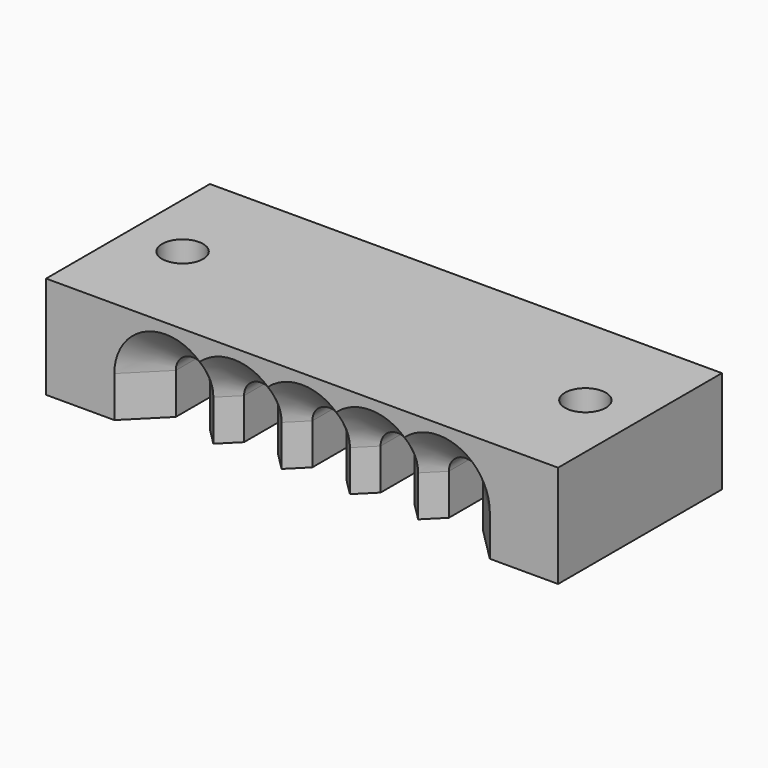
from build123d import *

# Parameters (mm, degrees)
F1_DEPTH     = 30
F3_D         = 6
F4_T1_DEPTH  = 18.8584149398
F4_T4_ANGLE  = 180
F4_T6_ANGLE  = 180
F4_T8_ANGLE  = 180
F4_T10_ANGLE = 180
F4_T12_ANGLE = 180


# Not quite as in the source:
# - a fillet or chamfer that OpenCascade refuses, or shapes differently, is made with other operations: its cross-section is extruded or revolved along the edge and cut away or added


with BuildPart() as f1:
    # F0 (on Front) → F1 (new body)
    with BuildSketch(Plane.XZ):
        with BuildLine():
            Line((29.6215080619, 22.2534802178), (-45.3784919381, 22.2534802178))
            Line((-45.3784919381, 22.2534802178), (-45.3784919381, 7.2534802178))
            Line((-45.3784919381, 7.2534802178), (-30.3784919381, 7.2534802178))
            Line((-30.3784919381, 7.2534802178), (-30.3784919381, 13.2534802178))
            ThreePointArc((-30.3784919381, 13.2534802178), (-27.8784919381, 15.7534802178), (-25.3784919381, 13.2534802178))
            Line((-25.3784919381, 13.2534802178), (-25.3784919381, 7.2534802178))
            Line((-25.3784919381, 7.2534802178), (-20.3784919381, 7.2534802178))
            Line((-20.3784919381, 7.2534802178), (-20.3784919381, 13.2534802178))
            ThreePointArc((-20.3784919381, 13.2534802178), (-17.8784919381, 15.7534802178), (-15.3784919381, 13.2534802178))
            Line((-15.3784919381, 13.2534802178), (-15.3784919381, 7.2534802178))
            Line((-15.3784919381, 7.2534802178), (-10.3784919381, 7.2534802178))
            Line((-10.3784919381, 7.2534802178), (-10.3784919381, 13.2534802178))
            ThreePointArc((-10.3784919381, 13.2534802178), (-7.8784919381, 15.7534802178), (-5.3784919381, 13.2534802178))
            Line((-5.3784919381, 13.2534802178), (-5.3784919381, 7.2534802178))
            Line((-5.3784919381, 7.2534802178), (-0.3784919381, 7.2534802178))
            Line((-0.3784919381, 7.2534802178), (-0.3784919381, 13.2534802178))
            ThreePointArc((-0.3784919381, 13.2534802178), (2.1215080619, 15.7534802178), (4.6215080619, 13.2534802178))
            Line((4.6215080619, 13.2534802178), (4.6215080619, 7.2534802178))
            Line((4.6215080619, 7.2534802178), (9.6215080619, 7.2534802178))
            Line((9.6215080619, 7.2534802178), (9.6215080619, 13.2534802178))
            ThreePointArc((9.6215080619, 13.2534802178), (12.1215080619, 15.7534802178), (14.6215080619, 13.2534802178))
            Line((14.6215080619, 13.2534802178), (14.6215080619, 7.2534802178))
            Line((14.6215080619, 7.2534802178), (29.6215080619, 7.2534802178))
            Line((29.6215080619, 7.2534802178), (29.6215080619, 22.2534802178))
        make_face()
    extrude(amount=F1_DEPTH)

    # F3 (through all)
    with Locations(Plane.XY.offset(22.2534802178)):
        with Locations((-37.3784919381, -15), (21.6215080619, -15)):
            Hole(F3_D / 2)

    # F4: chamfer of 5 on 5 edges, made by hand

    # F4_s2 → F4_t1 (cut)
    with BuildSketch(Plane.XY.offset(-5.604934722)):
        Polygon((-35.3784919381, -30), (-30.3784919381, -25), (-30.3784919381, -30), align=None)
        Polygon((-25.3784919381, -30), (-20.3784919381, -25), (-20.3784919381, -30), align=None)
        Polygon((-15.3784919381, -30), (-10.3784919381, -25), (-10.3784919381, -30), align=None)
        Polygon((-5.3784919381, -30), (-0.3784919381, -25), (-0.3784919381, -30), align=None)
        Polygon((4.6215080619, -30), (9.6215080619, -25), (9.6215080619, -30), align=None)
        Polygon((19.6215080619, -30), (14.6215080619, -25), (14.6215080619, -30), align=None)
        Polygon((9.6215080619, -30), (4.6215080619, -25), (4.6215080619, -30), align=None)
        Polygon((-0.3784919381, -30), (-5.3784919381, -25), (-5.3784919381, -30), align=None)
        Polygon((-10.3784919381, -30), (-15.3784919381, -25), (-15.3784919381, -30), align=None)
        Polygon((-20.3784919381, -30), (-25.3784919381, -25), (-25.3784919381, -30), align=None)
    extrude(amount=F4_T1_DEPTH, mode=Mode.SUBTRACT)

    # F4_s3 → F4_t4 (revolve, cut)
    with BuildSketch(Plane.XY.offset(13.2534802178)):
        Polygon((4.6215080619, -30), (9.6215080619, -25), (9.6215080619, -30), align=None)
    revolve(axis=Axis((12.1215080619, -30, 13.2534802178), (0, 1, 0)), revolution_arc=F4_T4_ANGLE, mode=Mode.SUBTRACT)

    # F4_s5 → F4_t6 (revolve, cut)
    with BuildSketch(Plane.XY.offset(13.2534802178)):
        Polygon((-5.3784919381, -30), (-0.3784919381, -25), (-0.3784919381, -30), align=None)
    revolve(axis=Axis((2.1215080619, -30, 13.2534802178), (0, 1, 0)), revolution_arc=F4_T6_ANGLE, mode=Mode.SUBTRACT)

    # F4_s7 → F4_t8 (revolve, cut)
    with BuildSketch(Plane.XY.offset(13.2534802178)):
        Polygon((-15.3784919381, -30), (-10.3784919381, -25), (-10.3784919381, -30), align=None)
    revolve(axis=Axis((-7.8784919381, -30, 13.2534802178), (0, 1, 0)), revolution_arc=F4_T8_ANGLE, mode=Mode.SUBTRACT)

    # F4_s9 → F4_t10 (revolve, cut)
    with BuildSketch(Plane.XY.offset(13.2534802178)):
        Polygon((-25.3784919381, -30), (-20.3784919381, -25), (-20.3784919381, -30), align=None)
    revolve(axis=Axis((-17.8784919381, -30, 13.2534802178), (0, 1, 0)), revolution_arc=F4_T10_ANGLE, mode=Mode.SUBTRACT)

    # F4_s11 → F4_t12 (revolve, cut)
    with BuildSketch(Plane.XY.offset(13.2534802178)):
        Polygon((-35.3784919381, -30), (-30.3784919381, -25), (-30.3784919381, -30), align=None)
    revolve(axis=Axis((-27.8784919381, -30, 13.2534802178), (0, 1, 0)), revolution_arc=F4_T12_ANGLE, mode=Mode.SUBTRACT)


solid = f1.part
